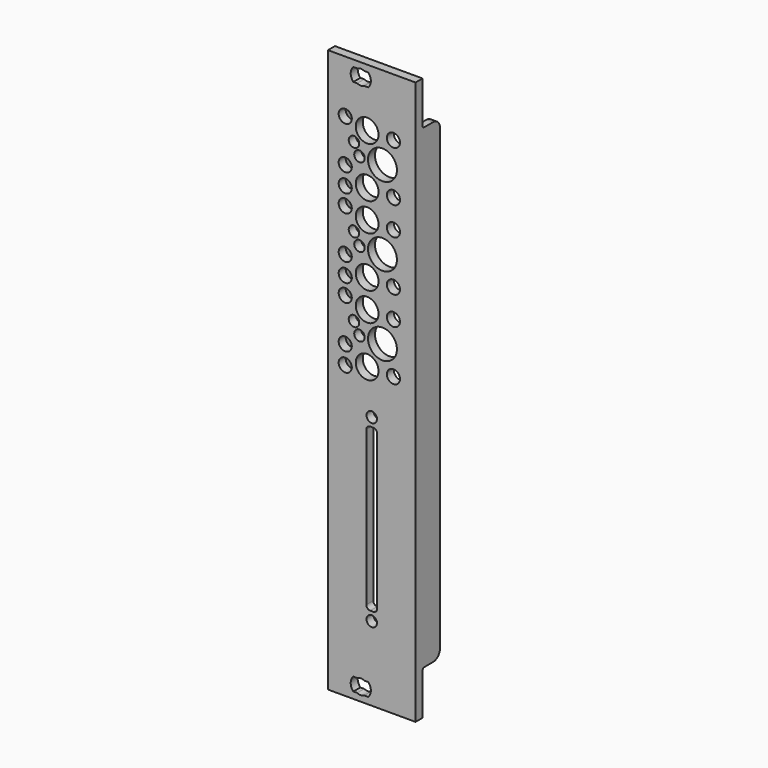
from build123d import *

# Parameters (mm, degrees)
F0_R     = 1.2
F0_R_2   = 1.500002
F0_R_3   = 2.6
F0_R_4   = 3.300001
F1_DEPTH = 2
F2_W     = 1.5
F2_H     = 108.500022
F3_DEPTH = 7
F4_R     = 2
F5_R     = 0.5


# Not quite as in the source:
# - ends of sketch curves that miss each other by under 0.0002 mm in the source are joined


with BuildPart() as f1:
    # F0 (on Front) → F1 (new body)
    with BuildSketch(Plane.XZ):
        Polygon((9.925, 64.250011), (-10.075, 64.250011), (-10.075, -61.250012), (-10.075, -64.250011), (9.925, -64.250011), align=None)
        with BuildLine():
            ThreePointArc((-3.375001, -59.75), (-2.5749995588, -59.549998), (-1.7749982215, -59.7500004152))
            Line((-1.7749982215, -59.7500004152), (-0.875001, -59.75))
            ThreePointArc((-0.875001, -59.75), (-0.275, -61.25), (-0.8750011748, -62.7499988335))
            Line((-0.8750011748, -62.7499988335), (-1.774999, -62.749999))
            ThreePointArc((-1.774999, -62.749999), (-2.5749995588, -62.950001), (-3.375001, -62.749999))
            Line((-3.375001, -62.749999), (-4.274999, -62.749999))
            ThreePointArc((-4.274999, -62.749999), (-4.875, -61.25), (-4.2749988252, -59.7500011665))
            Line((-4.2749988252, -59.7500011665), (-3.375001, -59.75))
        make_face(mode=Mode.SUBTRACT)
        with Locations((-0.074997, -47.24999)):
            Circle(F0_R, mode=Mode.SUBTRACT)
        with BuildLine():
            ThreePointArc((-1.325, -9.14999), (-1.0613958102, -8.5135931898), (-0.424999, -8.249989))
            Line((-0.424999, -8.249989), (0.274999, -8.249989))
            ThreePointArc((0.274999, -8.249989), (0.9113958102, -8.5135931898), (1.175, -9.14999))
            Line((1.175, -9.14999), (1.175, -26.74999))
            Line((1.175, -26.74999), (1.175, -44.34999))
            ThreePointArc((1.175, -44.34999), (0.9113958102, -44.9863868102), (0.274999, -45.249991))
            Line((0.274999, -45.249991), (-0.424999, -45.249991))
            ThreePointArc((-0.424999, -45.249991), (-1.0613958102, -44.9863868102), (-1.325, -44.34999))
            Line((-1.325, -44.34999), (-1.325, -26.74999))
            Line((-1.325, -26.74999), (-1.325, -9.14999))
        make_face(mode=Mode.SUBTRACT)
        with Locations((-0.074997, -6.24999)):
            Circle(F0_R, mode=Mode.SUBTRACT)
        with Locations((-6.125008, 2.249922)):
            Circle(F0_R_2, mode=Mode.SUBTRACT)
        with Locations((-6.125008, 6.499923)):
            Circle(F0_R_2, mode=Mode.SUBTRACT)
        with Locations((-6.125008, 16.249921)):
            Circle(F0_R_2, mode=Mode.SUBTRACT)
        with Locations((-6.125008, 20.249893)):
            Circle(F0_R_2, mode=Mode.SUBTRACT)
        with Locations((-6.125008, 24.499895)):
            Circle(F0_R_2, mode=Mode.SUBTRACT)
        with Locations((-4.125007, 11.74992)):
            Circle(F0_R, mode=Mode.SUBTRACT)
        with Locations((-2.875012, 9.24992)):
            Circle(F0_R, mode=Mode.SUBTRACT)
        with Locations((-1.12501, 3.499919)):
            Circle(F0_R_3, mode=Mode.SUBTRACT)
        with Locations((-1.12501, 14.999919)):
            Circle(F0_R_3, mode=Mode.SUBTRACT)
        with Locations((-4.125007, 29.749892)):
            Circle(F0_R, mode=Mode.SUBTRACT)
        with Locations((-2.875012, 27.249892)):
            Circle(F0_R, mode=Mode.SUBTRACT)
        with Locations((-1.12501, 21.499891)):
            Circle(F0_R_3, mode=Mode.SUBTRACT)
        with Locations((-6.125008, 34.249893)):
            Circle(F0_R_2, mode=Mode.SUBTRACT)
        with Locations((-6.125008, 38.249865)):
            Circle(F0_R_2, mode=Mode.SUBTRACT)
        with Locations((-6.125008, 42.499866)):
            Circle(F0_R_2, mode=Mode.SUBTRACT)
        with Locations((-6.125008, 52.249865)):
            Circle(F0_R_2, mode=Mode.SUBTRACT)
        with Locations((-4.125007, 47.749864)):
            Circle(F0_R, mode=Mode.SUBTRACT)
        with Locations((-2.875012, 45.249864)):
            Circle(F0_R, mode=Mode.SUBTRACT)
        with Locations((-1.12501, 32.999891)):
            Circle(F0_R_3, mode=Mode.SUBTRACT)
        with Locations((-1.12501, 39.499862)):
            Circle(F0_R_3, mode=Mode.SUBTRACT)
        with Locations((-1.12501, 50.999862)):
            Circle(F0_R_3, mode=Mode.SUBTRACT)
        with BuildLine():
            ThreePointArc((-3.3750014152, 62.7500117785), (-2.5749995588, 62.950014), (-1.7749978062, 62.7500113633))
            Line((-1.7749978062, 62.7500113633), (-0.875001, 62.750011))
            ThreePointArc((-0.875001, 62.750011), (-0.275, 61.250012), (-0.8750011748, 59.7500131665))
            Line((-0.8750011748, 59.7500131665), (-1.774999, 59.750012))
            ThreePointArc((-1.774999, 59.750012), (-2.5749995588, 59.55001), (-3.375001, 59.750012))
            Line((-3.375001, 59.750012), (-4.274999, 59.750012))
            ThreePointArc((-4.274999, 59.750012), (-4.875, 61.250012), (-4.2749988252, 62.7500108335))
            Line((-4.2749988252, 62.7500108335), (-3.3750014152, 62.7500117785))
        make_face(mode=Mode.SUBTRACT)
        with Locations((2.374988, 9.249948)):
            Circle(F0_R_4, mode=Mode.SUBTRACT)
        with Locations((4.874988, 3.499919)):
            Circle(F0_R_2, mode=Mode.SUBTRACT)
        with Locations((4.874988, 14.999919)):
            Circle(F0_R_2, mode=Mode.SUBTRACT)
        with Locations((2.374988, 27.24992)):
            Circle(F0_R_4, mode=Mode.SUBTRACT)
        with Locations((4.874988, 21.499891)):
            Circle(F0_R_2, mode=Mode.SUBTRACT)
        with Locations((2.374988, 45.249891)):
            Circle(F0_R_4, mode=Mode.SUBTRACT)
        with Locations((4.874988, 32.999891)):
            Circle(F0_R_2, mode=Mode.SUBTRACT)
        with Locations((4.874988, 39.499862)):
            Circle(F0_R_2, mode=Mode.SUBTRACT)
        with Locations((4.874988, 50.999862)):
            Circle(F0_R_2, mode=Mode.SUBTRACT)
    extrude(amount=F1_DEPTH)

    # F2 (on face) → F3 (join)
    with BuildSketch(Plane.XZ.offset(2)):
        with Locations((-9.325, 0)):
            Rectangle(F2_W, F2_H)
        with Locations((9.175, 0)):
            Rectangle(F2_W, F2_H)
    extrude(amount=-F3_DEPTH)

    # F4
    f4_edges = [f1.edges().sort_by_distance(p)[0] for p in [
        (-9.325, 5, 54.250011),
        (9.175, 5, 54.250011),
        (-9.325, 5, -54.250011),
        (9.175, 5, -54.250011),
    ]]
    fillet(f4_edges, radius=F4_R)

    # F5
    f5_edges = [f1.edges().sort_by_distance(p)[0] for p in [
        (9.175, 0, -54.250011),
        (-9.325, 0, -54.250011),
        (9.175, 0, 54.250011),
        (-9.325, 0, 54.250011),
    ]]
    fillet(f5_edges, radius=F5_R)


solid = f1.part
